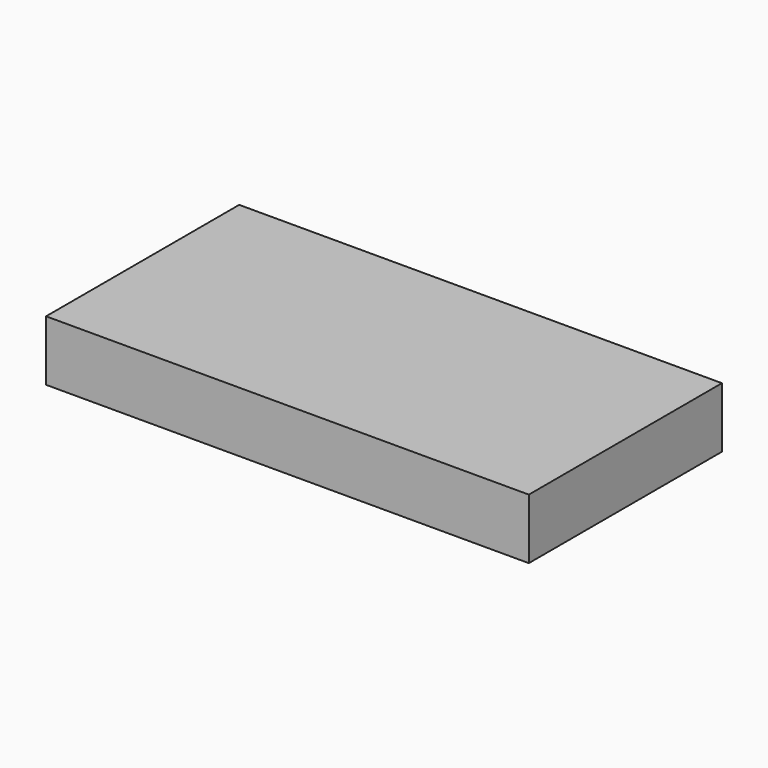
from build123d import *

# Parameters (mm, degrees)
F1_W     = 50.8
F1_H     = 12.7
F2_DEPTH = 101.6


# Not quite as in the source:
# - a variable given as a bare number and used for a length is read in inches; the dataset says mm whatever the document's units were


with BuildPart() as f2:
    # F1 (on Right) → F2 (new body)
    with BuildSketch(Plane.YZ):
        with Locations((25.4, -6.35)):
            Rectangle(F1_W, F1_H)
    extrude(amount=-F2_DEPTH)


solid = f2.part
